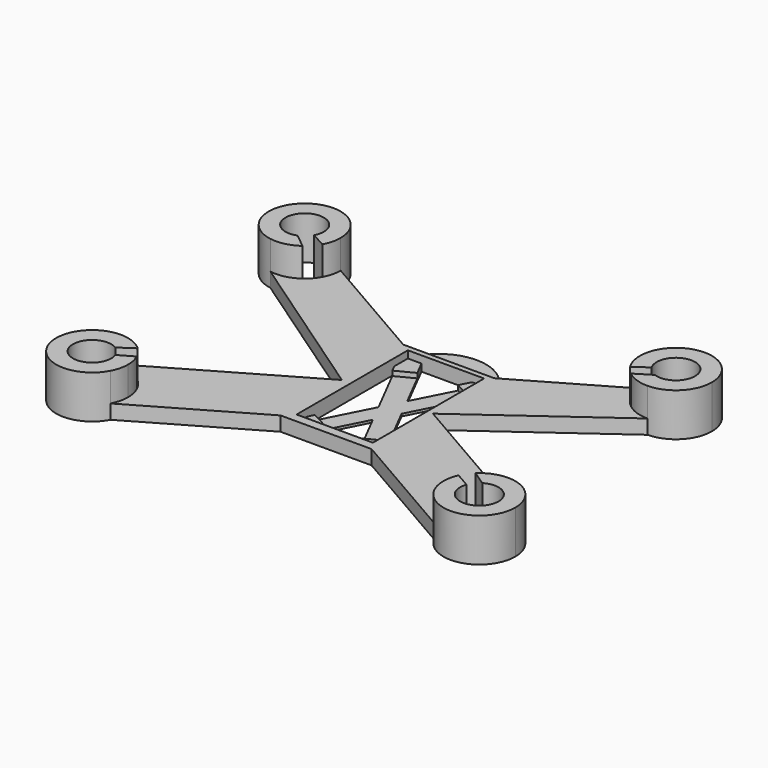
from build123d import *

# Parameters (mm, degrees)
F1_DEPTH = 3.81
F2_DEPTH = 11.43
F3_DEPTH = 1.905
F4_DEPTH = 0.635
F5_DEPTH = 0.381


with BuildPart() as f1:
    # F0 (on Top) → F1 (new body)
    with BuildSketch(Plane.XY):
        with BuildLine():
            Line((0, 40.64), (0, 20.32))
            Line((0, 20.32), (36.0270839263, 46.3555857197))
            ThreePointArc((36.0270839263, 46.3555857197), (32.7743226286, 46.8899395332), (29.8984857282, 48.5010112824))
            ThreePointArc((29.8984857282, 48.5010112824), (28.8184538619, 49.5338980727), (27.9132711745, 50.7230020447))
            ThreePointArc((27.9132711745, 50.7230020447), (26.7835232138, 53.1922797151), (26.3964543073, 55.88))
            Line((26.3964543073, 55.88), (0, 40.64))
        make_face()
        with BuildLine():
            Line((0, 20.32), (0, 0))
            Line((0, 0), (30.7958633586, -17.78))
            ThreePointArc((30.7958633586, -17.78), (29.7012441826, -13.6075167511), (30.5594271825, -9.3800672195))
            ThreePointArc((30.5594271825, -9.3800672195), (31.4801291394, -7.7913902048), (32.6885555919, -6.4088952646))
            ThreePointArc((32.6885555919, -6.4088952646), (38.1196995449, -3.8785721663), (43.9872077535, -5.0919175595))
            Line((43.9872077535, -5.0919175595), (0, 20.32))
        make_face()
        with BuildLine():
            Line((-54.9258633586, -17.78), (-24.13, 0))
            Line((-24.13, 0), (-24.13, 20.32))
            Line((-24.13, 20.32), (-68.1172077535, -5.0919175595))
            ThreePointArc((-68.1172077535, -5.0919175595), (-62.2496995449, -3.8785721663), (-56.8185555919, -6.4088952646))
            ThreePointArc((-56.8185555919, -6.4088952646), (-55.6101291394, -7.7913902048), (-54.6894271825, -9.3800672195))
            ThreePointArc((-54.6894271825, -9.3800672195), (-54.0454560084, -11.3134252867), (-53.8274732111, -13.3395190133))
            ThreePointArc((-53.8274732111, -13.3395190133), (-54.1061473504, -15.6266751246), (-54.9258633586, -17.78))
        make_face()
        with BuildLine():
            Line((-66.0401488201, 49.028525317), (-24.13, 20.32))
            Line((-24.13, 20.32), (-24.13, 40.64))
            Line((-24.13, 40.64), (-54.9258633586, 58.42))
            ThreePointArc((-54.9258633586, 58.42), (-55.2263237646, 56.0465016792), (-56.1087492964, 53.8227445173))
            ThreePointArc((-56.1087492964, 53.8227445173), (-57.3142816625, 52.1116859071), (-58.8644308605, 50.7052480957))
            ThreePointArc((-58.8644308605, 50.7052480957), (-62.2835733625, 49.1448461429), (-66.0401488201, 49.028525317))
        make_face()
        Polygon((-24.13, 0), (0, 0), (0, 20.32), (0, 40.64), (-24.13, 40.64), (-24.13, 20.32), align=None)
        Polygon((-18.3272082359, 2.3950056639), (-21.7771697789, 2.3950056639), (-21.7771697789, 5.8912090026), (-21.7771697789, 34.7188413143), (-21.7771697789, 39.2318554223), (-18.1576330215, 39.2318554223), (-4.7612613998, 39.2318554223), (-1.5657880576, 39.2318554223), (-1.5657880576, 35.2370127553), (-1.5657880576, 6.7390808836), (-1.5657880576, 2.3950056639), (-5.2699861117, 2.3950056639), align=None, mode=Mode.SUBTRACT)
    extrude(amount=F1_DEPTH)

    # F0 (on Top) → F2 (join)
    with BuildSketch(Plane.XY):
        with BuildLine():
            ThreePointArc((30.5594271825, -9.3800672195), (29.7012441826, -13.6075167511), (30.7958633586, -17.78))
            ThreePointArc((30.7958633586, -17.78), (41.5096293224, -22.585844874), (48.7474732111, -13.3395190133))
            ThreePointArc((48.7474732111, -13.3395190133), (47.4720102137, -8.5781364156), (43.9872077535, -5.0919175595))
            ThreePointArc((43.9872077535, -5.0919175595), (38.1196995449, -3.8785721663), (32.6885555919, -6.4088952646))
            Line((32.6885555919, -6.4088952646), (36.5475066082, -9.0208440228))
            ThreePointArc((36.5475066082, -9.0208440228), (41.6940688149, -8.9013194717), (44.3024732111, -13.3395190133))
            ThreePointArc((44.3024732111, -13.3395190133), (38.3505482132, -18.3441315655), (34.4417854953, -11.6215478365))
            Line((34.4417854953, -11.6215478365), (30.5594271825, -9.3800672195))
        make_face()
        with BuildLine():
            ThreePointArc((-68.1172077535, -5.0919175595), (-69.9554416118, -20.2043885167), (-54.9258633586, -17.78))
            ThreePointArc((-54.9258633586, -17.78), (-54.1061473504, -15.6266751246), (-53.8274732111, -13.3395190133))
            ThreePointArc((-53.8274732111, -13.3395190133), (-54.0454560084, -11.3134252867), (-54.6894271825, -9.3800672195))
            Line((-54.6894271825, -9.3800672195), (-58.5717854953, -11.6215478365))
            ThreePointArc((-58.5717854953, -11.6215478365), (-58.3478606589, -12.4675940154), (-58.2724732111, -13.3395190133))
            ThreePointArc((-58.2724732111, -13.3395190133), (-67.7906727527, -15.8111146171), (-60.6775066082, -9.0208440228))
            Line((-60.6775066082, -9.0208440228), (-56.8185555919, -6.4088952646))
            ThreePointArc((-56.8185555919, -6.4088952646), (-62.2496995449, -3.8785721663), (-68.1172077535, -5.0919175595))
        make_face()
        with BuildLine():
            ThreePointArc((-54.9258633586, 58.42), (-70.5985328755, 65.6954233217), (-66.0401488201, 49.028525317))
            ThreePointArc((-66.0401488201, 49.028525317), (-62.2835733625, 49.1448461429), (-58.8644308605, 50.7052480957))
            Line((-58.8644308605, 50.7052480957), (-62.5780124602, 53.6978363526))
            ThreePointArc((-62.5780124602, 53.6978363526), (-68.6532723441, 61.2741476343), (-59.3708633586, 58.42))
            ThreePointArc((-59.3708633586, 58.42), (-59.5311595199, 57.153937545), (-60.0019319176, 55.9677746772))
            Line((-60.0019319176, 55.9677746772), (-56.1087492964, 53.8227445173))
            ThreePointArc((-56.1087492964, 53.8227445173), (-55.2263237646, 56.0465016792), (-54.9258633586, 58.42))
        make_face()
        with BuildLine():
            ThreePointArc((29.8984857282, 48.5010112824), (32.7743226286, 46.8899395332), (36.0270839263, 46.3555857197))
            ThreePointArc((36.0270839263, 46.3555857197), (42.6938891398, 49.1822577357), (45.4464543073, 55.88))
            ThreePointArc((45.4464543073, 55.88), (35.9214543073, 65.405), (26.3964543073, 55.88))
            ThreePointArc((26.3964543073, 55.88), (26.7835232138, 53.1922797151), (27.9132711745, 50.7230020447))
            Line((27.9132711745, 50.7230020447), (31.5300523665, 53.3261814877))
            ThreePointArc((31.5300523665, 53.3261814877), (34.598941899, 60.7848303671), (41.0014543073, 55.88))
            ThreePointArc((41.0014543073, 55.88), (38.820808345, 51.708651757), (34.1510030615, 51.1184978855))
            Line((34.1510030615, 51.1184978855), (29.8984857282, 48.5010112824))
        make_face()
    extrude(amount=F2_DEPTH)

    # F0 (on Top) → F3 (join)
    with BuildSketch(Plane.XY):
        Polygon((-21.7771697789, 5.8912090026), (-21.7771697789, 2.3950056639), (-18.3272082359, 2.3950056639), (-16.8476979102, 5.2939299848), (-21.0003481494, 7.4132984911), align=None)
        Polygon((-6.7851137214, 5.3618797736), (-5.2699861117, 2.3950056639), (-1.5657880576, 2.3950056639), (-1.5657880576, 6.7390808836), (-2.0874397167, 7.760661653), align=None)
        Polygon((-21.7771697789, 39.2318554223), (-21.7771697789, 34.7188413143), (-20.8961134896, 32.993585252), (-16.1974461672, 35.3931075525), (-18.1576330215, 39.2318554223), align=None)
        Polygon((-2.074527, 34.2401993722), (-1.5657880576, 35.2370127553), (-1.5657880576, 39.2318554223), (-4.7612613998, 39.2318554223), (-6.2271772392, 36.3595678785), align=None)
    extrude(amount=F3_DEPTH)

    # F0 (on Top) → F4 (join)
    with BuildSketch(Plane.XY):
        Polygon((-21.0003481494, 7.4132984911), (-16.8476979102, 5.2939299848), (-11.8006188508, 15.1830804564), (-6.7851137214, 5.3618797736), (-2.0874397167, 7.760661653), (-8.8398640982, 20.9843268631), (-2.074527, 34.2401993722), (-6.2271772392, 36.3595678785), (-11.4576985252, 26.110984206), (-16.1974461672, 35.3931075525), (-20.8961134896, 32.993585252), (-14.41858046, 20.309488601), align=None)
    extrude(amount=F4_DEPTH)

    # F0 (on Top) → F5 (join)
    with BuildSketch(Plane.XY):
        with BuildLine():
            Line((-24.13, 40.64), (0, 40.64))
            ThreePointArc((0, 40.64), (-12.065, 49.8591743067), (-24.13, 40.64))
        make_face()
    extrude(amount=F5_DEPTH)


solid = f1.part
